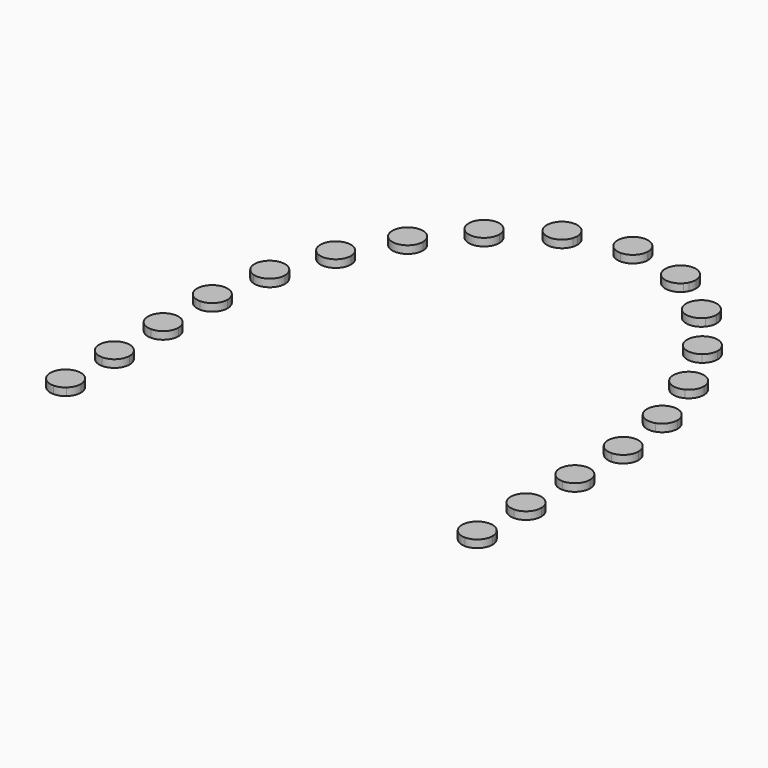
from build123d import *

# Parameters (mm, degrees)
F1_DEPTH = 1


with BuildPart() as f1:
    # F0 (on Top) → F1 (new body)
    with BuildSketch(Plane.XY):
        with BuildLine():
            ThreePointArc((-27, -22.2710574513), (-27.6273003349, -21.4879565386), (-28.2318954775, -20.6871959856))
            ThreePointArc((-28.2318954775, -20.6871959856), (-28.8909188329, -22.914249847), (-27, -24.2627700182))
            Line((-27, -24.2627700182), (-27, -22.2710574513))
        make_face()
        with BuildLine():
            ThreePointArc((-27, -24.2627700182), (-26.2996906188, -24.1361537938), (-25.6880517673, -23.7723367888))
            ThreePointArc((-25.6880517673, -23.7723367888), (-26.3547179775, -23.0310407999), (-27, -22.2710574513))
            Line((-27, -22.2710574513), (-27, -24.2627700182))
        make_face()
        with BuildLine():
            ThreePointArc((-27, -22.2710574513), (-26.3547179775, -23.0310407999), (-25.6880517673, -23.7723367888))
            ThreePointArc((-25.6880517673, -23.7723367888), (-25.1801241161, -23.0922588773), (-25, -22.2627700182))
            ThreePointArc((-25, -22.2627700182), (-25.5857864376, -20.8485564558), (-27, -20.2627700182))
            Line((-27, -20.2627700182), (-27, -22.2710574513))
        make_face()
        with BuildLine():
            ThreePointArc((-27, -20.2627700182), (-27.6514798288, -20.3718511853), (-28.2318954775, -20.6871959856))
            ThreePointArc((-28.2318954775, -20.6871959856), (-27.6273003349, -21.4879565386), (-27, -22.2710574513))
            Line((-27, -22.2710574513), (-27, -20.2627700182))
        make_face()
    extrude(amount=F1_DEPTH)


with BuildPart() as f1b:
    # F0 (on Top) → F1, piece 2 (new body)
    with BuildSketch(Plane.XY):
        with BuildLine():
            ThreePointArc((-27, -12.2627700182), (-29, -14.2627700182), (-27, -16.2627700182))
            Line((-27, -16.2627700182), (-27, -12.2627700182))
        make_face()
        with BuildLine():
            Line((-27, -12.2627700182), (-27, -16.2627700182))
            ThreePointArc((-27, -16.2627700182), (-25.5857864376, -15.6769835806), (-25, -14.2627700182))
            ThreePointArc((-25, -14.2627700182), (-25.5857864376, -12.8485564558), (-27, -12.2627700182))
        make_face()
    extrude(amount=F1_DEPTH)


with BuildPart() as f1c:
    # F0 (on Top) → F1, piece 3 (new body)
    with BuildSketch(Plane.XY):
        with BuildLine():
            Line((-27, -4.2627700182), (-27, -8.2627700182))
            ThreePointArc((-27, -8.2627700182), (-25.5857864376, -7.6769835806), (-25, -6.2627700182))
            ThreePointArc((-25, -6.2627700182), (-25.5857864376, -4.8485564558), (-27, -4.2627700182))
        make_face()
        with BuildLine():
            ThreePointArc((-27, -4.2627700182), (-29, -6.2627700182), (-27, -8.2627700182))
            Line((-27, -8.2627700182), (-27, -4.2627700182))
        make_face()
    extrude(amount=F1_DEPTH)


with BuildPart() as f1d:
    # F0 (on Top) → F1, piece 4 (new body)
    with BuildSketch(Plane.XY):
        with BuildLine():
            ThreePointArc((-26.9130430815, 3.7366593954), (-28.9547786194, 1.7805832958), (-27, -0.2623944974))
            Line((-27, -0.2623944974), (-27, 2.1762e-06))
            add(Edge.make_bspline(
                [(-26.9130430815, 3.7366593954), (-26.9557223388, 3.1632457962), (-27.0178727185, 1.9174252072), (-27.018694794, 0.6711028041), (-27, 2.1762e-06)],
                knots=[46.3026951197, 46.3026951197, 46.3026951197, 46.3026951197, 48.0262708445, 50.0404462243, 50.0404462243, 50.0404462243, 50.0404462243], degree=3))
        make_face()
        with BuildLine():
            Line((-27, 2.1762e-06), (-27, -0.2623944974))
            ThreePointArc((-27, -0.2623944974), (-25.5569482732, 0.3071577202), (-24.9552512695, 1.7371048277))
            ThreePointArc((-24.9552512695, 1.7371048277), (-25.5261927725, 3.1363159669), (-26.9130430815, 3.7366593954))
            add(Edge.make_bspline(
                [(-26.9130430815, 3.7366593954), (-26.9557223388, 3.1632457962), (-27.0178727185, 1.9174252072), (-27.018694794, 0.6711028041), (-27, 2.1762e-06)],
                knots=[46.3026951197, 46.3026951197, 46.3026951197, 46.3026951197, 48.0262708445, 50.0404462243, 50.0404462243, 50.0404462243, 50.0404462243], degree=3))
        make_face()
    extrude(amount=F1_DEPTH)


with BuildPart() as f1e:
    # F0 (on Top) → F1, piece 5 (new body)
    with BuildSketch(Plane.XY):
        with BuildLine():
            ThreePointArc((-23.7431047524, 9.6447404302), (-24.2093483136, 10.9283257161), (-25.3906959388, 11.6134476273))
            add(Edge.make_bspline(
                [(-25.3906959388, 11.6134476273), (-25.7772926058, 10.3391469136), (-26.1108947944, 9.0492772718), (-26.3697171129, 7.7454360971)],
                knots=[38.2700182558, 38.2700182558, 38.2700182558, 38.2700182558, 42.2565390205, 42.2565390205, 42.2565390205, 42.2565390205], degree=3))
            ThreePointArc((-26.3697171129, 7.7454360971), (-24.571188527, 8.0240577467), (-23.7431047524, 9.6447404302))
        make_face()
        with BuildLine():
            add(Edge.make_bspline(
                [(-25.3906959388, 11.6134476273), (-25.7772926058, 10.3391469136), (-26.1108947944, 9.0492772718), (-26.3697171129, 7.7454360971)],
                knots=[38.2700182558, 38.2700182558, 38.2700182558, 38.2700182558, 42.2565390205, 42.2565390205, 42.2565390205, 42.2565390205], degree=3))
            ThreePointArc((-25.3906959388, 11.6134476273), (-27.6819640036, 10.135479469), (-26.3697171129, 7.7454360971))
        make_face()
    extrude(amount=F1_DEPTH)


with BuildPart() as f1f:
    # F0 (on Top) → F1, piece 6 (new body)
    with BuildSketch(Plane.XY):
        with BuildLine():
            ThreePointArc((-21.1543015859, 17.2142911543), (-21.5173265672, 18.3633397991), (-22.4746143741, 19.0952550811))
            add(Edge.make_bspline(
                [(-22.4746143741, 19.0952550811), (-23.0556600273, 17.8981688231), (-23.5857836353, 16.6765500861), (-24.0685145965, 15.4354672251)],
                knots=[30.2406883205, 30.2406883205, 30.2406883205, 30.2406883205, 34.2317341084, 34.2317341084, 34.2317341084, 34.2317341084], degree=3))
            ThreePointArc((-24.0685145965, 15.4354672251), (-22.1122905546, 15.5071845347), (-21.1543015859, 17.2142911543))
        make_face()
        with BuildLine():
            add(Edge.make_bspline(
                [(-22.4746143741, 19.0952550811), (-23.0556600273, 17.8981688231), (-23.5857836353, 16.6765500861), (-24.0685145965, 15.4354672251)],
                knots=[30.2406883205, 30.2406883205, 30.2406883205, 30.2406883205, 34.2317341084, 34.2317341084, 34.2317341084, 34.2317341084], degree=3))
            ThreePointArc((-22.4746143741, 19.0952550811), (-24.9879488735, 18.0128759178), (-24.0685145965, 15.4354672251))
        make_face()
    extrude(amount=F1_DEPTH)


with BuildPart() as f1g:
    # F0 (on Top) → F1, piece 7 (new body)
    with BuildSketch(Plane.XY):
        with BuildLine():
            ThreePointArc((-17.3371352018, 24.244884358), (-17.609078729, 25.2517710581), (-18.3509560286, 25.9848414374))
            add(Edge.make_bspline(
                [(-18.3509560286, 25.9848414374), (-18.4580562206, 25.8374406972), (-19.2338042958, 24.7553116944), (-19.9604613575, 23.6396881807), (-20.5503087889, 22.6548498151)],
                knots=[22.2089072466, 22.2089072466, 22.2089072466, 22.2089072466, 22.7543847852, 26.1951280926, 26.1951280926, 26.1951280926, 26.1951280926], degree=3))
            ThreePointArc((-20.5503087889, 22.6548498151), (-18.4501028389, 22.4523516283), (-17.3371352018, 24.244884358))
        make_face()
        with BuildLine():
            add(Edge.make_bspline(
                [(-18.3509560286, 25.9848414374), (-18.4580562206, 25.8374406972), (-19.2338042958, 24.7553116944), (-19.9604613575, 23.6396881807), (-20.5503087889, 22.6548498151)],
                knots=[22.2089072466, 22.2089072466, 22.2089072466, 22.2089072466, 22.7543847852, 26.1951280926, 26.1951280926, 26.1951280926, 26.1951280926], degree=3))
            ThreePointArc((-18.3509560286, 25.9848414374), (-21.0059948925, 25.3471127068), (-20.5503087889, 22.6548498151))
        make_face()
    extrude(amount=F1_DEPTH)


with BuildPart() as f1h:
    # F0 (on Top) → F1, piece 8 (new body)
    with BuildSketch(Plane.XY):
        with BuildLine():
            add(Edge.make_bspline(
                [(-12.9074879803, 31.9008660262), (-13.4295174599, 31.4690091957), (-14.4233333877, 30.5803022949), (-15.3506230563, 29.6249489161), (-15.7914707556, 29.1417933074)],
                knots=[14.160331002, 14.160331002, 14.160331002, 14.160331002, 16.189226149, 18.1494166154, 18.1494166154, 18.1494166154, 18.1494166154], degree=3))
            ThreePointArc((-15.7914707556, 29.1417933074), (-13.5749506396, 28.5458585701), (-12.2579257305, 30.4256311694))
            ThreePointArc((-12.2579257305, 30.4256311694), (-12.4275056284, 31.2315854174), (-12.9074879803, 31.9008660262))
        make_face()
        with BuildLine():
            ThreePointArc((-13.5184707003, 32.2839116268), (-14.85169368, 31.6926993933), (-16.1591290831, 31.0464578861))
            ThreePointArc((-16.1591290831, 31.0464578861), (-16.2216749237, 30.0465677102), (-15.7914707556, 29.1417933074))
            add(Edge.make_bspline(
                [(-12.9074879803, 31.9008660262), (-13.4295174599, 31.4690091957), (-14.4233333877, 30.5803022949), (-15.3506230563, 29.6249489161), (-15.7914707556, 29.1417933074)],
                knots=[14.160331002, 14.160331002, 14.160331002, 14.160331002, 16.189226149, 18.1494166154, 18.1494166154, 18.1494166154, 18.1494166154], degree=3))
            ThreePointArc((-12.9074879803, 31.9008660262), (-13.1955727094, 32.1201535383), (-13.5184707003, 32.2839116268))
        make_face()
        with BuildLine():
            ThreePointArc((-13.5184707003, 32.2839116268), (-15.1065939408, 32.2366425633), (-16.1591290831, 31.0464578861))
            ThreePointArc((-16.1591290831, 31.0464578861), (-14.85169368, 31.6926993933), (-13.5184707003, 32.2839116268))
        make_face()
    extrude(amount=F1_DEPTH)


with BuildPart() as f1i:
    # F0 (on Top) → F1, piece 9 (new body)
    with BuildSketch(Plane.XY):
        with BuildLine():
            ThreePointArc((-5.8682321833, 34.504548266), (-7.565990037, 34.1724420368), (-9.2452641692, 33.7568524961))
            ThreePointArc((-9.2452641692, 33.7568524961), (-7.3415639248, 33.1588022784), (-5.8682321833, 34.504548266))
        make_face()
        with BuildLine():
            ThreePointArc((-9.5710208071, 34.233800808), (-9.4254503771, 33.9835053297), (-9.2452641692, 33.7568524961))
            ThreePointArc((-9.2452641692, 33.7568524961), (-7.565990037, 34.1724420368), (-5.8682321833, 34.504548266))
            ThreePointArc((-5.8682321833, 34.504548266), (-5.7976283907, 34.8043879181), (-5.7739062126, 35.111513252))
            ThreePointArc((-5.7739062126, 35.111513252), (-5.8211522845, 35.543661486), (-5.9606583088, 35.9553924134))
            add(Edge.make_bspline(
                [(-5.9606583088, 35.9553924134), (-6.4328058861, 35.777718689), (-7.6644782169, 35.2625574752), (-8.8531185259, 34.6509988525), (-9.5710208071, 34.233800808)],
                knots=[6.0884535184, 6.0884535184, 6.0884535184, 6.0884535184, 7.6012051941, 10.089797983, 10.089797983, 10.089797983, 10.089797983], degree=3))
        make_face()
        with BuildLine():
            ThreePointArc((-5.9606583088, 35.9553924134), (-8.6347398115, 36.9167737636), (-9.5710208071, 34.233800808))
            add(Edge.make_bspline(
                [(-5.9606583088, 35.9553924134), (-6.4328058861, 35.777718689), (-7.6644782169, 35.2625574752), (-8.8531185259, 34.6509988525), (-9.5710208071, 34.233800808)],
                knots=[6.0884535184, 6.0884535184, 6.0884535184, 6.0884535184, 7.6012051941, 10.089797983, 10.089797983, 10.089797983, 10.089797983], degree=3))
        make_face()
    extrude(amount=F1_DEPTH)


with BuildPart() as f1j:
    # F0 (on Top) → F1, piece 10 (new body)
    with BuildSketch(Plane.XY):
        with BuildLine():
            ThreePointArc((2, 37), (-0.0345949994, 38.9997007741), (-1.998803186, 36.9308203529))
            add(Edge.make_bspline(
                [(0, 37), (-0.2833414452, 37.0069688983), (-0.9504816494, 37.0068654793), (-1.6172669927, 36.9687119393), (-1.998803186, 36.9308203529)],
                knots=[0, 0, 0, 0, 0.8506820357, 2.0004209479, 2.0004209479, 2.0004209479, 2.0004209479], degree=3))
            add(Edge.make_bspline(
                [(0, 37), (0.2833414452, 37.0069688983), (0.9504816494, 37.0068654793), (1.6172669927, 36.9687119393), (1.998803186, 36.9308203529)],
                knots=[0, 0, 0, 0, 0.8506820357, 2.0004209479, 2.0004209479, 2.0004209479, 2.0004209479], degree=3))
            ThreePointArc((1.998803186, 36.9308203529), (1.9997007741, 36.9654050006), (2, 37))
        make_face()
        with BuildLine():
            ThreePointArc((-1.998803186, 36.9308203529), (-1.389539619, 35.5615356636), (0, 35))
            ThreePointArc((0, 35), (1.389539619, 35.5615356636), (1.998803186, 36.9308203529))
            add(Edge.make_bspline(
                [(0, 37), (0.2833414452, 37.0069688983), (0.9504816494, 37.0068654793), (1.6172669927, 36.9687119393), (1.998803186, 36.9308203529)],
                knots=[0, 0, 0, 0, 0.8506820357, 2.0004209479, 2.0004209479, 2.0004209479, 2.0004209479], degree=3))
            add(Edge.make_bspline(
                [(0, 37), (-0.2833414452, 37.0069688983), (-0.9504816494, 37.0068654793), (-1.6172669927, 36.9687119393), (-1.998803186, 36.9308203529)],
                knots=[0, 0, 0, 0, 0.8506820357, 2.0004209479, 2.0004209479, 2.0004209479, 2.0004209479], degree=3))
        make_face()
    extrude(amount=F1_DEPTH)


with BuildPart() as f1k:
    # F0 (on Top) → F1, piece 11 (new body)
    with BuildSketch(Plane.XY):
        with BuildLine():
            add(Edge.make_bspline(
                [(5.9606583088, 35.9553924134), (6.4328058861, 35.777718689), (7.6644782169, 35.2625574752), (8.8531185259, 34.6509988525), (9.5710208071, 34.233800808)],
                knots=[6.0884535184, 6.0884535184, 6.0884535184, 6.0884535184, 7.6012051941, 10.089797983, 10.089797983, 10.089797983, 10.089797983], degree=3))
            ThreePointArc((9.5710208071, 34.233800808), (9.7225248501, 34.6610852271), (9.7739062126, 35.111513252))
            ThreePointArc((9.7739062126, 35.111513252), (8.2060544466, 37.0642671801), (5.9606583088, 35.9553924134))
        make_face()
        with BuildLine():
            ThreePointArc((5.8682321833, 34.504548266), (7.565990037, 34.1724420368), (9.2452641692, 33.7568524961))
            ThreePointArc((9.2452641692, 33.7568524961), (9.4254503771, 33.9835053297), (9.5710208071, 34.233800808))
            add(Edge.make_bspline(
                [(5.9606583088, 35.9553924134), (6.4328058861, 35.777718689), (7.6644782169, 35.2625574752), (8.8531185259, 34.6509988525), (9.5710208071, 34.233800808)],
                knots=[6.0884535184, 6.0884535184, 6.0884535184, 6.0884535184, 7.6012051941, 10.089797983, 10.089797983, 10.089797983, 10.089797983], degree=3))
            ThreePointArc((5.9606583088, 35.9553924134), (5.7779522374, 35.2386656362), (5.8682321833, 34.504548266))
        make_face()
        with BuildLine():
            ThreePointArc((5.8682321833, 34.504548266), (7.3415639248, 33.1588022784), (9.2452641692, 33.7568524961))
            ThreePointArc((9.2452641692, 33.7568524961), (7.565990037, 34.1724420368), (5.8682321833, 34.504548266))
        make_face()
    extrude(amount=F1_DEPTH)


with BuildPart() as f1l:
    # F0 (on Top) → F1, piece 12 (new body)
    with BuildSketch(Plane.XY):
        with BuildLine():
            ThreePointArc((16.2579257305, 30.4256311694), (16.2330721435, 30.7399505093), (16.1591290831, 31.0464578861))
            ThreePointArc((16.1591290831, 31.0464578861), (14.85169368, 31.6926993933), (13.5184707003, 32.2839116268))
            ThreePointArc((13.5184707003, 32.2839116268), (13.1955727094, 32.1201535383), (12.9074879803, 31.9008660262))
            add(Edge.make_bspline(
                [(12.9074879803, 31.9008660262), (13.4295174599, 31.4690091957), (14.4233333877, 30.5803022949), (15.3506230563, 29.6249489161), (15.7914707556, 29.1417933074)],
                knots=[14.160331002, 14.160331002, 14.160331002, 14.160331002, 16.189226149, 18.1494166154, 18.1494166154, 18.1494166154, 18.1494166154], degree=3))
            ThreePointArc((15.7914707556, 29.1417933074), (16.1376983298, 29.7426560785), (16.2579257305, 30.4256311694))
        make_face()
        with BuildLine():
            add(Edge.make_bspline(
                [(12.9074879803, 31.9008660262), (13.4295174599, 31.4690091957), (14.4233333877, 30.5803022949), (15.3506230563, 29.6249489161), (15.7914707556, 29.1417933074)],
                knots=[14.160331002, 14.160331002, 14.160331002, 14.160331002, 16.189226149, 18.1494166154, 18.1494166154, 18.1494166154, 18.1494166154], degree=3))
            ThreePointArc((12.9074879803, 31.9008660262), (12.8753547069, 28.9804677307), (15.7914707556, 29.1417933074))
        make_face()
        with BuildLine():
            ThreePointArc((13.5184707003, 32.2839116268), (14.85169368, 31.6926993933), (16.1591290831, 31.0464578861))
            ThreePointArc((16.1591290831, 31.0464578861), (15.1065939408, 32.2366425633), (13.5184707003, 32.2839116268))
        make_face()
    extrude(amount=F1_DEPTH)


with BuildPart() as f1m:
    # F0 (on Top) → F1, piece 13 (new body)
    with BuildSketch(Plane.XY):
        with BuildLine():
            ThreePointArc((21.3371352018, 24.244884358), (20.3440219019, 25.9729408309), (18.3509560286, 25.9848414374))
            add(Edge.make_bspline(
                [(18.3509560286, 25.9848414374), (18.4580562206, 25.8374406972), (19.2338042958, 24.7553116944), (19.9604613575, 23.6396881807), (20.5503087889, 22.6548498151)],
                knots=[22.2089072466, 22.2089072466, 22.2089072466, 22.2089072466, 22.7543847852, 26.1951280926, 26.1951280926, 26.1951280926, 26.1951280926], degree=3))
            ThreePointArc((20.5503087889, 22.6548498151), (21.1296679316, 23.3578519951), (21.3371352018, 24.244884358))
        make_face()
        with BuildLine():
            add(Edge.make_bspline(
                [(18.3509560286, 25.9848414374), (18.4580562206, 25.8374406972), (19.2338042958, 24.7553116944), (19.9604613575, 23.6396881807), (20.5503087889, 22.6548498151)],
                knots=[22.2089072466, 22.2089072466, 22.2089072466, 22.2089072466, 22.7543847852, 26.1951280926, 26.1951280926, 26.1951280926, 26.1951280926], degree=3))
            ThreePointArc((18.3509560286, 25.9848414374), (17.6682755112, 23.1426560093), (20.5503087889, 22.6548498151))
        make_face()
    extrude(amount=F1_DEPTH)


with BuildPart() as f1n:
    # F0 (on Top) → F1, piece 14 (new body)
    with BuildSketch(Plane.XY):
        with BuildLine():
            ThreePointArc((25.1543015859, 17.2142911543), (24.3033502307, 18.851266173), (22.4746143741, 19.0952550811))
            add(Edge.make_bspline(
                [(22.4746143741, 19.0952550811), (23.0556600273, 17.8981688231), (23.5857836353, 16.6765500861), (24.0685145965, 15.4354672251)],
                knots=[30.2406883205, 30.2406883205, 30.2406883205, 30.2406883205, 34.2317341084, 34.2317341084, 34.2317341084, 34.2317341084], degree=3))
            ThreePointArc((24.0685145965, 15.4354672251), (24.8614082055, 16.172280123), (25.1543015859, 17.2142911543))
        make_face()
        with BuildLine():
            add(Edge.make_bspline(
                [(22.4746143741, 19.0952550811), (23.0556600273, 17.8981688231), (23.5857836353, 16.6765500861), (24.0685145965, 15.4354672251)],
                knots=[30.2406883205, 30.2406883205, 30.2406883205, 30.2406883205, 34.2317341084, 34.2317341084, 34.2317341084, 34.2317341084], degree=3))
            ThreePointArc((22.4746143741, 19.0952550811), (21.3206542983, 16.4157063908), (24.0685145965, 15.4354672251))
        make_face()
    extrude(amount=F1_DEPTH)


with BuildPart() as f1o:
    # F0 (on Top) → F1, piece 15 (new body)
    with BuildSketch(Plane.XY):
        with BuildLine():
            add(Edge.make_bspline(
                [(25.3906959388, 11.6134476273), (25.7772926058, 10.3391469136), (26.1108947944, 9.0492772718), (26.3697171129, 7.7454360971)],
                knots=[38.2700182558, 38.2700182558, 38.2700182558, 38.2700182558, 42.2565390205, 42.2565390205, 42.2565390205, 42.2565390205], degree=3))
            ThreePointArc((26.3697171129, 7.7454360971), (27.3637874359, 8.4728242047), (27.7431047524, 9.6447404302))
            ThreePointArc((27.7431047524, 9.6447404302), (27.0266900384, 11.178496869), (25.3906959388, 11.6134476273))
        make_face()
        with BuildLine():
            ThreePointArc((25.3906959388, 11.6134476273), (23.8042455013, 9.1540013914), (26.3697171129, 7.7454360971))
            add(Edge.make_bspline(
                [(25.3906959388, 11.6134476273), (25.7772926058, 10.3391469136), (26.1108947944, 9.0492772718), (26.3697171129, 7.7454360971)],
                knots=[38.2700182558, 38.2700182558, 38.2700182558, 38.2700182558, 42.2565390205, 42.2565390205, 42.2565390205, 42.2565390205], degree=3))
        make_face()
    extrude(amount=F1_DEPTH)


with BuildPart() as f1p:
    # F0 (on Top) → F1, piece 16 (new body)
    with BuildSketch(Plane.XY):
        with BuildLine():
            Line((27, 2.1762e-06), (27, -0.2623944974))
            ThreePointArc((27, -0.2623944974), (28.3851983771, 0.3388018314), (28.9552512695, 1.7371048277))
            ThreePointArc((28.9552512695, 1.7371048277), (28.3544624087, 3.1661633248), (26.9130430815, 3.7366593954))
            add(Edge.make_bspline(
                [(26.9130430815, 3.7366593954), (26.9557223388, 3.1632457962), (27.0178727185, 1.9174252072), (27.018694794, 0.6711028041), (27, 2.1762e-06)],
                knots=[46.3026951197, 46.3026951197, 46.3026951197, 46.3026951197, 48.0262708445, 50.0404462243, 50.0404462243, 50.0404462243, 50.0404462243], degree=3))
        make_face()
        with BuildLine():
            ThreePointArc((26.9130430815, 3.7366593954), (24.9557239197, 1.6936263597), (27, -0.2623944974))
            Line((27, -0.2623944974), (27, 2.1762e-06))
            add(Edge.make_bspline(
                [(26.9130430815, 3.7366593954), (26.9557223388, 3.1632457962), (27.0178727185, 1.9174252072), (27.018694794, 0.6711028041), (27, 2.1762e-06)],
                knots=[46.3026951197, 46.3026951197, 46.3026951197, 46.3026951197, 48.0262708445, 50.0404462243, 50.0404462243, 50.0404462243, 50.0404462243], degree=3))
        make_face()
    extrude(amount=F1_DEPTH)


with BuildPart() as f1q:
    # F0 (on Top) → F1, piece 17 (new body)
    with BuildSketch(Plane.XY):
        with BuildLine():
            Line((27, -4.2627700182), (27, -8.2627700182))
            ThreePointArc((27, -8.2627700182), (28.4142135624, -7.6769835806), (29, -6.2627700182))
            ThreePointArc((29, -6.2627700182), (28.4142135624, -4.8485564558), (27, -4.2627700182))
        make_face()
        with BuildLine():
            ThreePointArc((27, -4.2627700182), (25, -6.2627700182), (27, -8.2627700182))
            Line((27, -8.2627700182), (27, -4.2627700182))
        make_face()
    extrude(amount=F1_DEPTH)


with BuildPart() as f1r:
    # F0 (on Top) → F1, piece 18 (new body)
    with BuildSketch(Plane.XY):
        with BuildLine():
            ThreePointArc((27, -12.2627700182), (25, -14.2627700182), (27, -16.2627700182))
            Line((27, -16.2627700182), (27, -12.2627700182))
        make_face()
        with BuildLine():
            Line((27, -12.2627700182), (27, -16.2627700182))
            ThreePointArc((27, -16.2627700182), (28.4142135624, -15.6769835806), (29, -14.2627700182))
            ThreePointArc((29, -14.2627700182), (28.4142135624, -12.8485564558), (27, -12.2627700182))
        make_face()
    extrude(amount=F1_DEPTH)


with BuildPart() as f1s:
    # F0 (on Top) → F1, piece 19 (new body)
    with BuildSketch(Plane.XY):
        with BuildLine():
            ThreePointArc((27, -20.2627700182), (25.1266162244, -21.562460637), (25.6880517673, -23.7723367888))
            ThreePointArc((25.6880517673, -23.7723367888), (26.3547179775, -23.0310407999), (27, -22.2710574513))
            Line((27, -22.2710574513), (27, -20.2627700182))
        make_face()
        with BuildLine():
            ThreePointArc((28.2318954775, -20.6871959856), (27.6273003349, -21.4879565386), (27, -22.2710574513))
            Line((27, -22.2710574513), (27, -24.2627700182))
            ThreePointArc((27, -24.2627700182), (28.4142135624, -23.6769835806), (29, -22.2627700182))
            ThreePointArc((29, -22.2627700182), (28.7977473342, -21.3863542935), (28.2318954775, -20.6871959856))
        make_face()
        with BuildLine():
            Line((27, -20.2627700182), (27, -22.2710574513))
            ThreePointArc((27, -22.2710574513), (27.6273003349, -21.4879565386), (28.2318954775, -20.6871959856))
            ThreePointArc((28.2318954775, -20.6871959856), (27.6514798288, -20.3718511853), (27, -20.2627700182))
        make_face()
        with BuildLine():
            ThreePointArc((27, -22.2710574513), (26.3547179775, -23.0310407999), (25.6880517673, -23.7723367888))
            ThreePointArc((25.6880517673, -23.7723367888), (26.2996906188, -24.1361537938), (27, -24.2627700182))
            Line((27, -24.2627700182), (27, -22.2710574513))
        make_face()
    extrude(amount=F1_DEPTH)


solid = Compound([f1.part, f1b.part, f1c.part, f1d.part, f1e.part, f1f.part, f1g.part, f1h.part, f1i.part, f1j.part, f1k.part, f1l.part, f1m.part, f1n.part, f1o.part, f1p.part, f1q.part, f1r.part, f1s.part])
